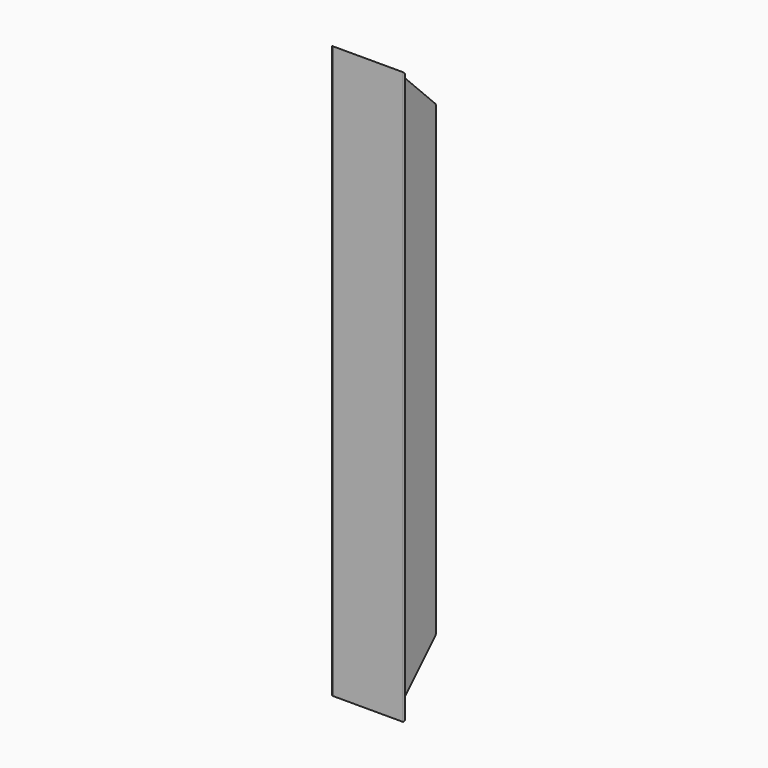
from build123d import *

# Parameters (mm, degrees)
F1_DEPTH = 153
F3_DEPTH = 30
F4_R     = 1
F6_R     = 0.5
F7_R     = 0.5


# Not quite as in the source:
# - two fillets or chamfers of one size are made in one step
# - a pattern or mirror of a feature is missing from the dataset's text; its kind, count and spacing are read off the source's solid


with BuildPart() as f1:
    # F0 (on Top) → F1 (new body, symmetric)
    with BuildSketch(Plane.XY):
        Polygon((-14, 0.5), (-17, 0.5), (-20, -2.5), (20, -2.5), (17, 0.5), (14, 0.5), (11, 0.5), (-11, 0.5), align=None)
        Polygon((-14, 25.5), (-14, 0.5), (-11, 0.5), (-11, 4), (-11, 7), (-11, 25.5), align=None)
        Polygon((11, 4), (11, 0.5), (14, 0.5), (14, 25.5), (11, 25.5), (11, 7), align=None)
        Polygon((-11, 7), (-11, 4), (-5, 4), (-5, 7), (-5, 15), (-8, 15), (-8, 7), align=None)
        Polygon((5, 4), (11, 4), (11, 7), (8, 7), (8, 15), (5, 15), (5, 7), align=None)
    extrude(amount=F1_DEPTH, both=True)

    # F2 (on Right) → F3 (cut, symmetric)
    with BuildSketch(Plane.YZ):
        Polygon((25.5, 153), (0.5, 153), (-2.5, 153), (25.5, 125), align=None)
    f3 = extrude(amount=F3_DEPTH, both=True, mode=Mode.SUBTRACT)

    # F3_copies: F3 across plane
    add(f3.mirror(Plane(origin=(0, 0, 0), x_dir=(-1, 0, 0), z_dir=(0, 0, -1))), mode=Mode.SUBTRACT)

    # F4
    f4_edges = [f1.edges().sort_by_distance(p)[0] for p in [
        (17, 0.5, 0),
        (12.5, 25.5, 125),
        (-11, 0.5, 0),
        (-12.5, 25.5, 125),
        (-17, 0.5, 0),
        (11, 0.5, 0),
        (6.5, 15, 135.5),
        (-6.5, 15, 135.5),
        (12.5, 25.5, -125),
        (6.5, 15, -135.5),
        (-6.5, 15, -135.5),
        (-12.5, 25.5, -125),
        (5, 4, 0),
        (-5, 4, 0),
    ]]
    fillet(f4_edges, radius=F4_R)

    # F6
    f6_edges = [f1.edges().sort_by_distance(p)[0] for p in [
        (-8, 7, 0),
        (-11, 7, 0),
        (-11, 4, 0),
        (11, 4, 0),
        (11, 7, 0),
        (8, 7, 0),
    ]]
    fillet(f6_edges, radius=F6_R)

    # F7
    f7_edges = [f1.edges().sort_by_distance(p)[0] for p in [
        (20, -2.5, 0),
        (-20, -2.5, 0),
    ]]
    fillet(f7_edges, radius=F7_R)


solid = f1.part
